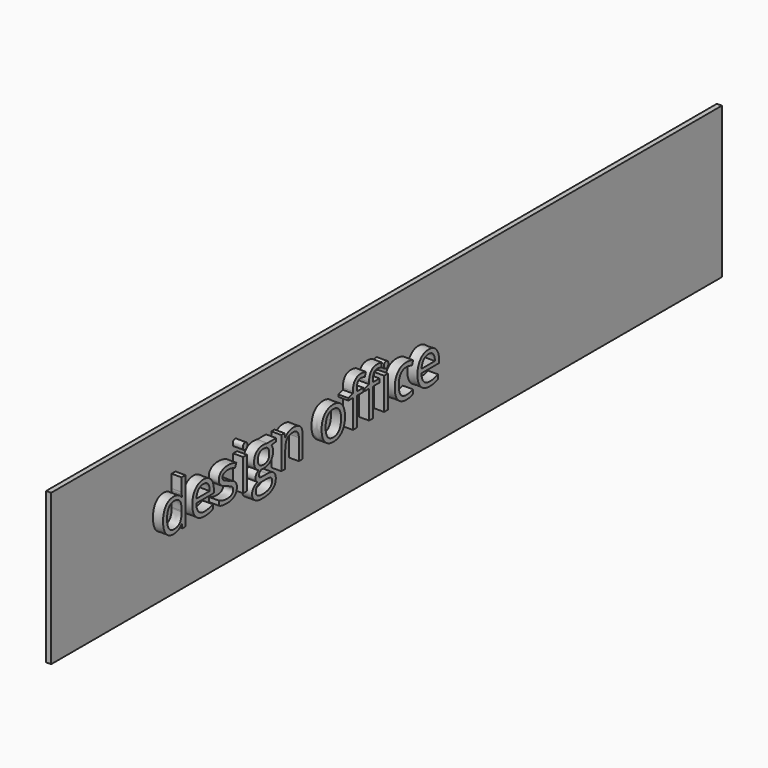
from build123d import *

# Parameters (mm, degrees)
F0_W         = 15
F0_H         = 450
F1_DEPTH     = 2500
F2_TEXT_SIZE = 177.6671244038
F3_DEPTH     = 30


# Not quite as in the source:
# - Text() gives the source's letters only with a copy of the font that has no kerning and outlines rounded to 1/6400 em; it was checked with that copy


with BuildPart() as f1:
    # F0 (on Front) → F1 (new body)
    with BuildSketch(Plane.XZ):
        with Locations((-2.7000385213, 225)):
            Rectangle(F0_W, F0_H)
    extrude(amount=F1_DEPTH)

    # F2 (on face) → F3 (join)
    with BuildSketch(Plane.YZ.offset(4.7999614787)):
        with Locations((-2130.2652359009, 182.7212274075)):
            Text('design office', F2_TEXT_SIZE, font='Open Sans', text_align=(TextAlign.LEFT, TextAlign.BOTTOM))
    extrude(amount=F3_DEPTH)


solid = f1.part
